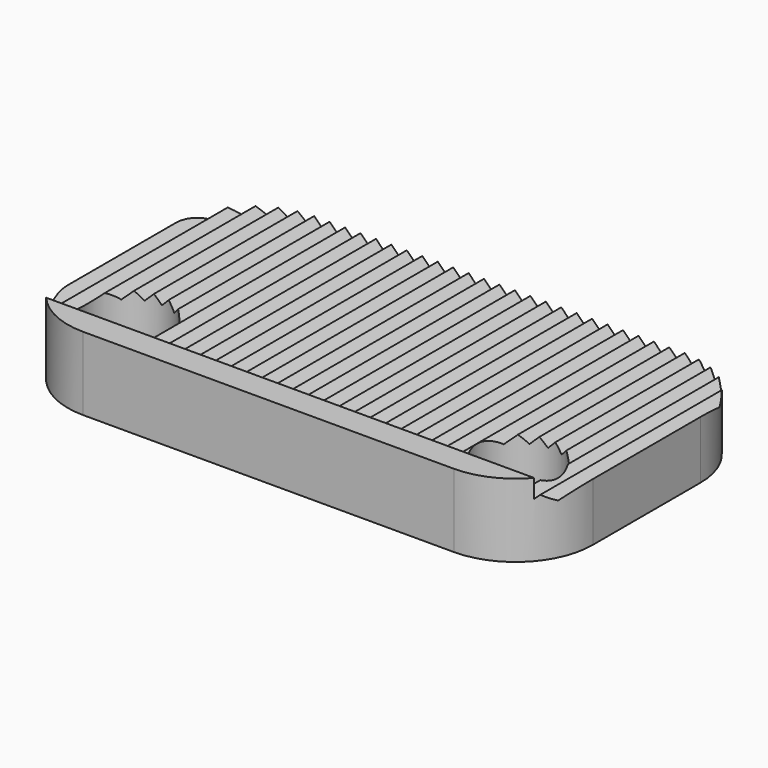
from build123d import *

# Parameters (mm, degrees)
F0_W        = 34.544
F0_H        = 19
F1_DEPTH    = 3.81
F3_R        = 2.667
F4_DEPTH    = 10.16
F6_DEPTH    = 19.001
F7_W        = 34.544
F7_H        = 1.778
F8_DEPTH    = 4.826
F9_T1_DEPTH = 30.226
F9_T3_DEPTH = 29.21


# Not quite as in the source:
# - a fillet or chamfer that OpenCascade refuses, or shapes differently, is made with other operations: its cross-section is extruded or revolved along the edge and cut away or added


with BuildPart() as f1:
    # F0 (on Top) → F1 (new body)
    with BuildSketch(Plane.XY):
        Rectangle(F0_W, F0_H)
    extrude(amount=F1_DEPTH)

    # F3 (on face) → F4 (cut)
    with BuildSketch(Plane.XY.offset(3.81)):
        with Locations((-12.827, -5.055)):
            Circle(F3_R)
        with Locations((12.827, -5.055)):
            Circle(F3_R)
    extrude(amount=-F4_DEPTH, mode=Mode.SUBTRACT)

    # F5 (on face) → F6 (cut, through all)
    with BuildSketch(Plane.XZ.offset(9.5)):
        Polygon((-17.78, 3.302), (-17.272, 3.81), (-18.288, 3.81), align=None)
        Polygon((-16.764, 3.302), (-16.256, 3.81), (-17.272, 3.81), align=None)
        Polygon((-15.748, 3.302), (-15.24, 3.81), (-16.256, 3.81), align=None)
        Polygon((-14.732, 3.302), (-14.224, 3.81), (-15.24, 3.81), align=None)
        Polygon((-13.716, 3.302), (-13.208, 3.81), (-14.224, 3.81), align=None)
        Polygon((-12.7, 3.302), (-12.192, 3.81), (-13.208, 3.81), align=None)
        Polygon((-11.684, 3.302), (-11.176, 3.81), (-12.192, 3.81), align=None)
        Polygon((-10.668, 3.302), (-10.16, 3.81), (-11.176, 3.81), align=None)
        Polygon((-9.652, 3.302), (-9.144, 3.81), (-10.16, 3.81), align=None)
        Polygon((-8.636, 3.302), (-8.128, 3.81), (-9.144, 3.81), align=None)
        Polygon((-7.62, 3.302), (-7.112, 3.81), (-8.128, 3.81), align=None)
        Polygon((-6.604, 3.302), (-6.096, 3.81), (-7.112, 3.81), align=None)
        Polygon((-5.588, 3.302), (-5.08, 3.81), (-6.096, 3.81), align=None)
        Polygon((-4.572, 3.302), (-4.064, 3.81), (-5.08, 3.81), align=None)
        Polygon((-3.556, 3.302), (-3.048, 3.81), (-4.064, 3.81), align=None)
        Polygon((-2.54, 3.302), (-2.032, 3.81), (-3.048, 3.81), align=None)
        Polygon((-1.524, 3.302), (-1.016, 3.81), (-2.032, 3.81), align=None)
        Polygon((-0.508, 3.302), (0, 3.81), (-1.016, 3.81), align=None)
        Polygon((0.508, 3.302), (1.016, 3.81), (0, 3.81), align=None)
        Polygon((1.524, 3.302), (2.032, 3.81), (1.016, 3.81), align=None)
        Polygon((2.54, 3.302), (3.048, 3.81), (2.032, 3.81), align=None)
        Polygon((3.556, 3.302), (4.064, 3.81), (3.048, 3.81), align=None)
        Polygon((4.572, 3.302), (5.08, 3.81), (4.064, 3.81), align=None)
        Polygon((5.588, 3.302), (6.096, 3.81), (5.08, 3.81), align=None)
        Polygon((6.604, 3.302), (7.112, 3.81), (6.096, 3.81), align=None)
        Polygon((7.62, 3.302), (8.128, 3.81), (7.112, 3.81), align=None)
        Polygon((8.636, 3.302), (9.144, 3.81), (8.128, 3.81), align=None)
        Polygon((9.652, 3.302), (10.16, 3.81), (9.144, 3.81), align=None)
        Polygon((10.668, 3.302), (11.176, 3.81), (10.16, 3.81), align=None)
        Polygon((11.684, 3.302), (12.192, 3.81), (11.176, 3.81), align=None)
        Polygon((12.7, 3.302), (13.208, 3.81), (12.192, 3.81), align=None)
        Polygon((13.716, 3.302), (14.224, 3.81), (13.208, 3.81), align=None)
        Polygon((14.732, 3.302), (15.24, 3.81), (14.224, 3.81), align=None)
        Polygon((15.748, 3.302), (16.256, 3.81), (15.24, 3.81), align=None)
        Polygon((16.764, 3.302), (17.272, 3.81), (16.256, 3.81), align=None)
    extrude(amount=-F6_DEPTH, mode=Mode.SUBTRACT)

    # F7 (on face) → F8 (join)
    with BuildSketch(Plane(origin=(0, 0, 0), x_dir=(1, 0, 0), z_dir=(0, 0, -1))):
        with Locations((0, 8.611)):
            Rectangle(F7_W, F7_H)
    extrude(amount=-F8_DEPTH)

    # F9: fillet of radius 5.08 on 4 edges, made by hand

    # F9_s2 → F9_t1 (cut)
    with BuildSketch(Plane.XY.offset(-12.7)):
        with BuildLine():
            ThreePointArc((12.192, -9.5), (15.7841024484, -8.0121024484), (17.272, -4.42))
            Line((17.272, -4.42), (17.272, -9.5))
            Line((17.272, -9.5), (12.192, -9.5))
        make_face()
        with BuildLine():
            ThreePointArc((-12.192, -9.5), (-15.7841024484, -8.0121024484), (-17.272, -4.42))
            Line((-17.272, -4.42), (-17.272, -9.5))
            Line((-17.272, -9.5), (-12.192, -9.5))
        make_face()
    extrude(amount=F9_T1_DEPTH, mode=Mode.SUBTRACT)

    # F9_s4 → F9_t3 (cut)
    with BuildSketch(Plane.XY.offset(-12.7)):
        with BuildLine():
            ThreePointArc((17.272, 4.42), (15.7841024484, 8.0121024484), (12.192, 9.5))
            Line((12.192, 9.5), (17.272, 9.5))
            Line((17.272, 9.5), (17.272, 4.42))
        make_face()
        with BuildLine():
            ThreePointArc((-12.192, 9.5), (-15.7841024484, 8.0121024484), (-17.272, 4.42))
            Line((-17.272, 4.42), (-17.272, 9.5))
            Line((-17.272, 9.5), (-12.192, 9.5))
        make_face()
    extrude(amount=F9_T3_DEPTH, mode=Mode.SUBTRACT)


solid = f1.part
